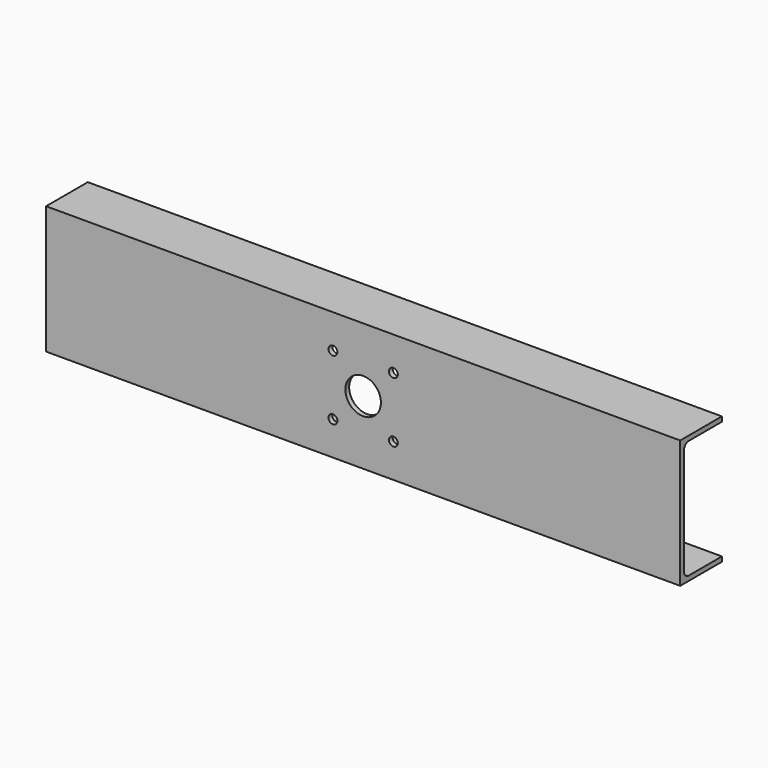
from build123d import *

# Parameters (mm, degrees)
F0_W        = 1070
F0_H        = 200
F1_DEPTH    = 80
F2_T        = 8
F3_T1_DEPTH = 1070
F4_D        = 60
F5_D        = 15


# Not quite as in the source:
# - a fillet or chamfer that OpenCascade refuses, or shapes differently, is made with other operations: its cross-section is extruded or revolved along the edge and cut away or added


with BuildPart() as f1:
    # F0 (on Front) → F1 (new body)
    with BuildSketch(Plane.XZ):
        Rectangle(F0_W, F0_H)
    extrude(amount=-F1_DEPTH)

    # F2
    f2_openings = [f1.faces().sort_by_distance(p)[0] for p in [
        (0, 80, 0),
        (535, 40, 0),
        (-535, 40, 0),
    ]]
    offset(amount=F2_T, openings=f2_openings, kind=Kind.INTERSECTION)

    # F3: fillet of radius 10 on 2 edges, made by hand

    # F3_s2 → F3_t1 (join)
    with BuildSketch(Plane.YZ.offset(-535)):
        with BuildLine():
            ThreePointArc((10, -100), (2.9289321881, -97.0710678119), (0, -90))
            Line((0, -90), (0, -100))
            Line((0, -100), (10, -100))
        make_face()
        with BuildLine():
            ThreePointArc((0, 90), (2.9289321881, 97.0710678119), (10, 100))
            Line((10, 100), (0, 100))
            Line((0, 100), (0, 90))
        make_face()
    extrude(amount=F3_T1_DEPTH)

    # F4 (through all)
    with Locations(Plane(origin=(0, 0, 0), x_dir=(1, 0, 0), z_dir=(0, 1, 0))):
        with Locations((0, 0)):
            Hole(F4_D / 2)

    # F5 (through all)
    with Locations(Plane(origin=(0, 0, 0), x_dir=(1, 0, 0), z_dir=(0, 1, 0))):
        with Locations((-51, -51), (51, -51), (51, 51), (-51, 51)):
            Hole(F5_D / 2)


solid = f1.part
